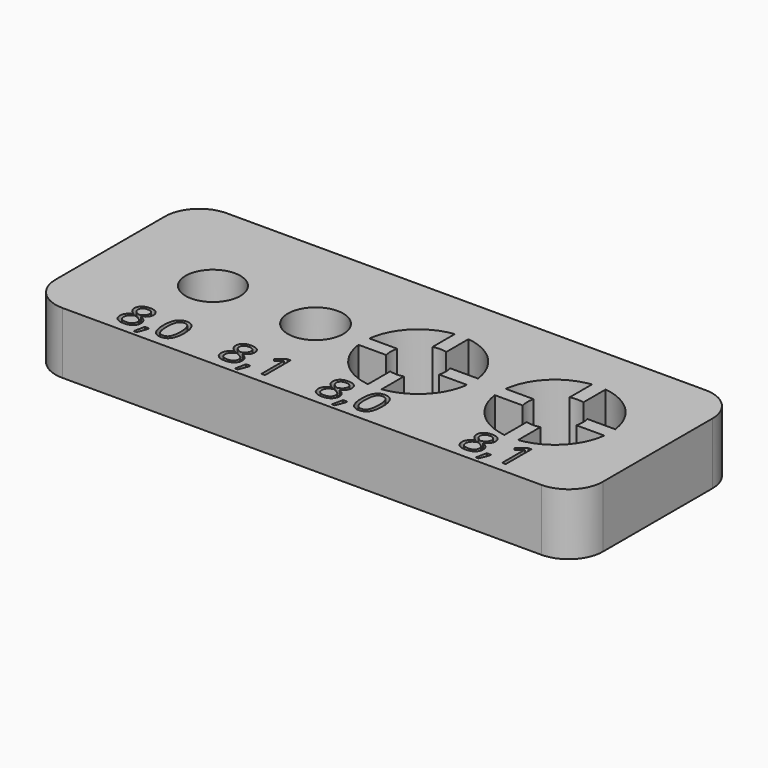
from build123d import *

# Parameters (mm, degrees)
F0_R         = 4
F0_R_2       = 4.05
F1_DEPTH     = 9
F2_TEXT_SIZE = 6.582404847
F3_DEPTH     = 1


# Not quite as in the source:
# - Text() gives the source's letters only with a copy of the font that has no kerning and outlines rounded to 1/6400 em; it was checked with that copy


with BuildPart() as f1:
    # F0 (on Top) → F1 (new body)
    with BuildSketch(Plane.XY):
        with BuildLine():
            Line((35, 15), (-35, 15))
            ThreePointArc((-35, 15), (-38.5355339059, 13.5355339059), (-40, 10))
            Line((-40, 10), (-40, -10))
            ThreePointArc((-40, -10), (-38.5355339059, -13.5355339059), (-35, -15))
            Line((-35, -15), (35, -15))
            ThreePointArc((35, -15), (38.5355339059, -13.5355339059), (40, -10))
            Line((40, -10), (40, 10))
            ThreePointArc((40, 10), (38.5355339059, 13.5355339059), (35, 15))
        make_face()
        with Locations((-25, 0)):
            Circle(F0_R, mode=Mode.SUBTRACT)
        with Locations((-10, 0)):
            Circle(F0_R_2, mode=Mode.SUBTRACT)
        with BuildLine():
            ThreePointArc((4, 3.8729833462), (5, 4), (6, 3.8729833462))
            Line((6, 3.8729833462), (6, 7.9372539332))
            ThreePointArc((6, 7.9372539332), (10.6568542495, 5.6568542495), (12.9372539332, 1))
            Line((12.9372539332, 1), (8.8729833462, 1))
            ThreePointArc((8.8729833462, 1), (9, 0), (8.8729833462, -1))
            Line((8.8729833462, -1), (12.9372539332, -1))
            ThreePointArc((12.9372539332, -1), (10.6568542495, -5.6568542495), (6, -7.9372539332))
            Line((6, -7.9372539332), (6, -3.8729833462))
            ThreePointArc((6, -3.8729833462), (5, -4), (4, -3.8729833462))
            Line((4, -3.8729833462), (4, -7.9372539332))
            ThreePointArc((4, -7.9372539332), (-0.6568542495, -5.6568542495), (-2.9372539332, -1))
            Line((-2.9372539332, -1), (1.1270166538, -1))
            ThreePointArc((1.1270166538, -1), (1, 0), (1.1270166538, 1))
            Line((1.1270166538, 1), (-2.9372539332, 1))
            ThreePointArc((-2.9372539332, 1), (-0.6568542495, 5.6568542495), (4, 7.9372539332))
            Line((4, 7.9372539332), (4, 3.8729833462))
        make_face(mode=Mode.SUBTRACT)
        with BuildLine():
            ThreePointArc((24, 3.9246018906), (25, 4.05), (26, 3.9246018906))
            Line((26, 3.9246018906), (26, 8))
            ThreePointArc((26, 8), (30.7008771255, 5.7008771255), (33, 1))
            Line((33, 1), (28.9246018906, 1))
            ThreePointArc((28.9246018906, 1), (29.05, 0), (28.9246018906, -1))
            Line((28.9246018906, -1), (33, -1))
            ThreePointArc((33, -1), (30.7008771255, -5.7008771255), (26, -8))
            Line((26, -8), (26, -3.9246018906))
            ThreePointArc((26, -3.9246018906), (25, -4.05), (24, -3.9246018906))
            Line((24, -3.9246018906), (24, -8))
            ThreePointArc((24, -8), (19.2991228745, -5.7008771255), (17, -1))
            Line((17, -1), (21.0753981094, -1))
            ThreePointArc((21.0753981094, -1), (20.95, 0), (21.0753981094, 1))
            Line((21.0753981094, 1), (17, 1))
            ThreePointArc((17, 1), (19.2991228745, 5.7008771255), (24, 8))
            Line((24, 8), (24, 3.9246018906))
        make_face(mode=Mode.SUBTRACT)
    extrude(amount=F1_DEPTH)

    # F2 (on face) → F3 (cut)
    with BuildSketch(Plane.XY.offset(9)):
        with Locations((-29.0485597281, -13.5355339059)):
            Text('8,0', F2_TEXT_SIZE, font='Open Sans', text_align=(TextAlign.LEFT, TextAlign.BOTTOM))
        with Locations((-14.2491148726, -13.5355339059)):
            Text('8,1', F2_TEXT_SIZE, font='Open Sans', text_align=(TextAlign.LEFT, TextAlign.BOTTOM))
        with Locations((-0.0712628341, -13.5355339059)):
            Text('8,0', F2_TEXT_SIZE, font='Open Sans', text_align=(TextAlign.LEFT, TextAlign.BOTTOM))
        with Locations((20.9464207292, -13.5355339059)):
            Text('8,1', F2_TEXT_SIZE, font='Open Sans', text_align=(TextAlign.LEFT, TextAlign.BOTTOM))
    extrude(amount=-F3_DEPTH, mode=Mode.SUBTRACT)


solid = f1.part
